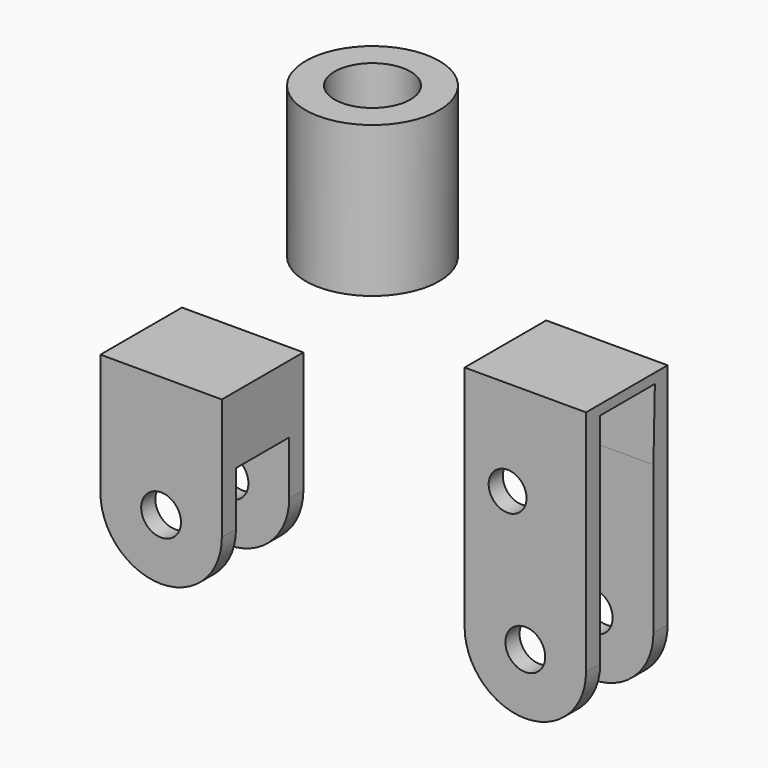
from build123d import *

# Parameters (mm, degrees)
F0_W     = 6.0325
F0_H     = 31.496
F0_R     = 4.1656
F2_DEPTH = 10.668
F0_R_2   = 3.9624
F3_W     = 13.9187620953
F3_H     = 16.6894979775
F4_DEPTH = 101.601
F5_DEPTH = 101.601


# Not quite as in the source:
# - the program builds the solid bodies; features that only make, move or delete a surface that nothing else refers to are left out


with BuildPart() as f1:
    # F0 (on Front) → F1 (revolve)
    with BuildSketch(Plane.XZ):
        with Locations((10.95375, 70.612)):
            Rectangle(F0_W, F0_H)
    revolve(axis=Axis((0, 0, 43.18), (0, 0, 1)))


with BuildPart() as f2:
    # F0 (on Front) → F2 (new body, symmetric)
    with BuildSketch(Plane.XZ):
        with BuildLine():
            ThreePointArc((-48.3905182989, 0), (-35.6905182989, 12.7), (-22.9905182989, 0))
            Line((-22.9905182989, 0), (-22.9905182989, 25.4))
            Line((-22.9905182989, 25.4), (-48.3905182989, 25.4))
            Line((-48.3905182989, 25.4), (-48.3905182989, 0))
        make_face()
        with BuildLine():
            ThreePointArc((-48.3905182989, 0), (-35.6905182989, -12.7), (-22.9905182989, 0))
            ThreePointArc((-22.9905182989, 0), (-35.6905182989, 12.7), (-48.3905182989, 0))
        make_face()
        with Locations((-35.6905182989, 0)):
            Circle(F0_R, mode=Mode.SUBTRACT)
    extrude(amount=F2_DEPTH, both=True)


with BuildPart() as f2b:
    # F0 (on Front) → F2, piece 2 (new body, symmetric)
    with BuildSketch(Plane.XZ):
        with BuildLine():
            ThreePointArc((27.8094817011, 0), (40.5094817011, 12.7), (53.2094817011, 0))
            Line((53.2094817011, 0), (53.2094817011, 47.8088483214))
            Line((53.2094817011, 47.8088483214), (27.8094817011, 47.8088483214))
            Line((27.8094817011, 47.8088483214), (27.8094817011, 0))
        make_face()
        with Locations((36.8013158441, 27.94)):
            Circle(F0_R_2, mode=Mode.SUBTRACT)
        with BuildLine():
            ThreePointArc((27.8094817011, 0), (40.5094817011, -12.7), (53.2094817011, 0))
            ThreePointArc((53.2094817011, 0), (40.5094817011, 12.7), (27.8094817011, 0))
        make_face()
        with BuildLine():
            ThreePointArc((44.6750817011, 0), (40.5094817011, -4.1656), (36.3438817011, 0))
            ThreePointArc((36.3438817011, 0), (40.5094817011, 4.1656), (44.6750817011, 0))
        make_face(mode=Mode.SUBTRACT)
    extrude(amount=F2_DEPTH, both=True)


with BuildPart() as f4_tool:
    # F3 (on face) → F4 (new body, through all)
    with BuildSketch(Plane.YZ.offset(53.2094817011)):
        with Locations((0, -8.3447489887)):
            Rectangle(F3_W, F3_H)
        Polygon((-6.9593810476, 0), (6.9593810476, 0), (6.9593810476, 11.2505020225), (-4.3954011053, 11.2505020225), (-6.9593810476, 11.2505020225), align=None)
        Polygon((-6.9593810476, 31.0145973873), (6.9593810476, 31.0145973873), (7.3419297114, 45.72), (-6.9593810476, 45.72), align=None)
    extrude(amount=-F4_DEPTH)


with BuildPart() as f2_1:
    add(f2.part)

    # F4: cut by f4_tool
    add(f4_tool.part, mode=Mode.SUBTRACT)


with BuildPart() as f2b_1:
    add(f2b.part)

    # F4: cut by f4_tool
    add(f4_tool.part, mode=Mode.SUBTRACT)

    # F3 (on face) → F5 (cut, through all)
    with BuildSketch(Plane.YZ.offset(53.2094817011)):
        with Locations((0, -8.3447489887)):
            Rectangle(F3_W, F3_H)
        Polygon((-4.3954011053, 11.2505020225), (6.9593810476, 11.2505020225), (6.9593810476, 31.0145973873), (-6.9593810476, 31.0145973873), (-6.9593810476, 11.2505020225), align=None)
    extrude(amount=-F5_DEPTH, mode=Mode.SUBTRACT)


solid = Compound([f1.part, f2_1.part, f2b_1.part])
